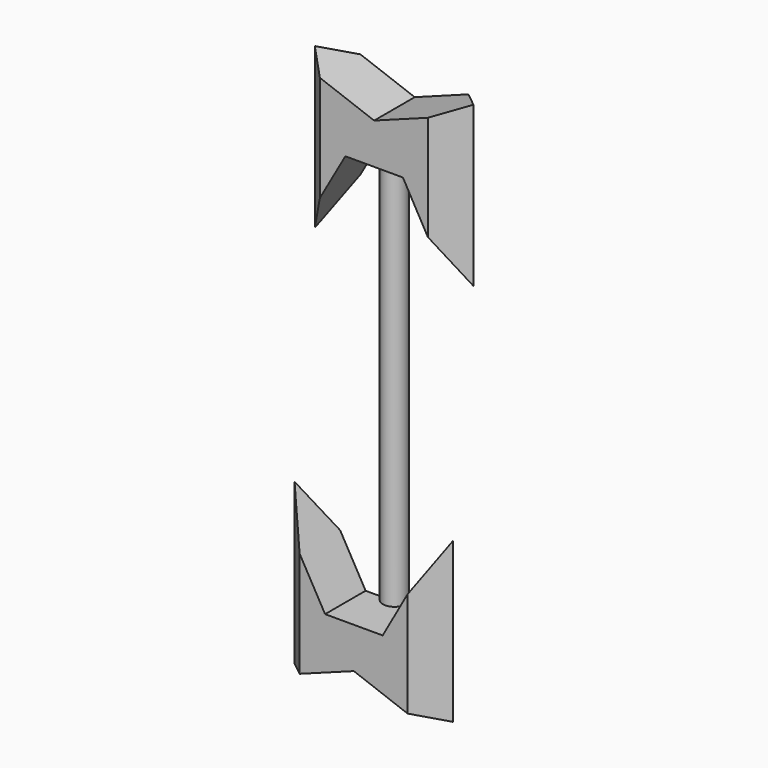
from build123d import *

# Parameters (mm, degrees)
F0_R        = 1.27
F1_DEPTH    = 43.18
F3_DEPTH    = 2.794
F4_T1_DEPTH = 48.6435811926
F5_DEPTH    = 5.588
F6_T1_DEPTH = 48.6435811926


# Not quite as in the source:
# - a fillet or chamfer that OpenCascade refuses, or shapes differently, is made with other operations: its cross-section is extruded or revolved along the edge and cut away or added


with BuildPart() as f1:
    # F0 (on Top) → F1 (new body)
    with BuildSketch(Plane.XY):
        Circle(F0_R)
    extrude(amount=F1_DEPTH)


with BuildPart() as f3:
    # F2 (on Front) → F3 (new body, symmetric)
    with BuildSketch(Plane.XZ):
        Polygon((-3.1743557192, 43.1767851114), (3.1734784134, 43.1767851114), (10.9989056364, 29.2393378913), (10.9989056364, 51.7546199262), (0, 47.6719401777), (-11.0619841143, 51.7546199262), (-11.0619841143, 29.2393378913), align=None)
    extrude(amount=F3_DEPTH, both=True)

    # F4: chamfer of 5.08 on 4 edges, made by hand

    # F4_s2 → F4_t1 (cut)
    with BuildSketch(Plane.XY.offset(16.1751883125)):
        Polygon((10.9989056364, 2.286), (5.9189056364, -2.794), (10.9989056364, -2.794), align=None)
        Polygon((10.9989056364, -2.286), (5.9189056364, 2.794), (10.9989056364, 2.794), align=None)
        Polygon((-11.0619841143, 2.286), (-5.9819841143, -2.794), (-11.0619841143, -2.794), align=None)
        Polygon((-11.0619841143, -2.286), (-5.9819841143, 2.794), (-11.0619841143, 2.794), align=None)
    extrude(amount=F4_T1_DEPTH, mode=Mode.SUBTRACT)


with BuildPart() as f5:
    # F2 (on Front) → F5 (new body)
    with BuildSketch(Plane.XZ):
        Polygon((10.9989056364, 13.8055048883), (3.1734784134, -0.1319423318), (-3.1743557192, -0.1319423318), (-11.0619841143, 13.8055048883), (-11.0619841143, -8.7097771466), (0, -4.627097398), (10.9989056364, -8.7097771466), align=None)
    extrude(amount=F5_DEPTH)

    # F6: chamfer of 5.08 on 4 edges, made by hand

    # F6_s2 → F6_t1 (cut)
    with BuildSketch(Plane.XY.offset(-21.7739267254)):
        Polygon((-11.0619841143, -5.08), (-5.9819841143, 0), (-11.0619841143, 0), align=None)
        Polygon((-11.0619841143, -0.508), (-5.9819841143, -5.588), (-11.0619841143, -5.588), align=None)
        Polygon((10.9989056364, -0.508), (5.9189056364, -5.588), (10.9989056364, -5.588), align=None)
        Polygon((10.9989056364, -5.08), (5.9189056364, 0), (10.9989056364, 0), align=None)
    extrude(amount=F6_T1_DEPTH, mode=Mode.SUBTRACT)


solid = Compound([f1.part, f3.part, f5.part])
